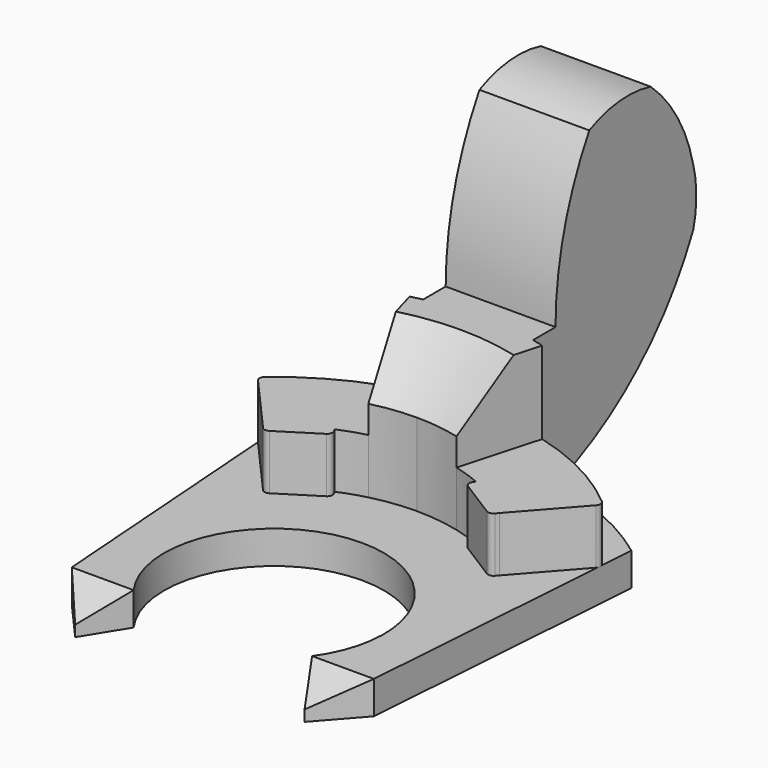
from build123d import *

# Parameters (mm, degrees)
F1_DEPTH    = 1.2
F3_DEPTH    = 12.5
F5_DEPTH    = 2
F6_DEPTH    = 5
F7_T2_ANGLE = 119.2786087223
F8_DEPTH    = 5
F10_DEPTH   = 4
F11_DEPTH   = 5


# Not quite as in the source:
# - a fillet or chamfer that OpenCascade refuses, or shapes differently, is made with other operations: its cross-section is extruded or revolved along the edge and cut away or added
# - a feature names something its author has since deleted; it is built from what else it names


with BuildPart() as f1:
    # F0 (on Top) → F1 (new body)
    with BuildSketch(Plane.XY):
        with BuildLine():
            ThreePointArc((-3.25, -2.3318447633), (0, 4), (3.25, -2.3318447633))
            Line((3.25, -2.3318447633), (4.1771243445, -3.8318447633))
            Line((4.1771243445, -3.8318447633), (5.5, -2.3318447633))
            Line((5.5, -2.3318447633), (6.2861850371, 8.4103434936))
            ThreePointArc((6.2861850371, 8.4103434936), (0, 10.5), (-6.2861850371, 8.4103434936))
            Line((-6.2861850371, 8.4103434936), (-5.5, -2.3318447633))
            Line((-5.5, -2.3318447633), (-4.1771243445, -3.8318447633))
            Line((-4.1771243445, -3.8318447633), (-3.25, -2.3318447633))
        make_face()
    extrude(amount=F1_DEPTH)

    # F2 (on Right) → F3 (cut, symmetric)
    with BuildSketch(Plane.YZ):
        Polygon((-3.8318447633, 0.4), (-2.3318447633, 1.2), (-3.8318447633, 1.2), align=None)
    extrude(amount=F3_DEPTH, both=True, mode=Mode.SUBTRACT)

    # F4 (on face) → F5 (join)
    with BuildSketch(Plane.XY.offset(1.2)):
        with BuildLine():
            Line((0, 9.4893432962), (0, 9.5))
            ThreePointArc((0, 9.5), (-1.0056504861, 9.4466219941), (-2, 9.2870878105))
            ThreePointArc((-2, 9.2870878105), (-2.207287093, 9.2400153511), (-2.4134691055, 9.1883168686))
            Line((-2.4134691055, 9.1883168686), (-1.6054997382, 6.2986006851))
            ThreePointArc((-1.6054997382, 6.2986006851), (-0.809041268, 6.4494536378), (0, 6.5))
            Line((0, 6.5), (0, 9.4893432962))
        make_face()
        with BuildLine():
            Line((0, 10.3126084432), (0, 9.5))
            ThreePointArc((0, 9.5), (1.0056504861, 9.4466219941), (2, 9.2870878105))
            Line((2, 9.2870878105), (2, 10.3126084432))
            Line((2, 10.3126084432), (0, 10.3126084432))
        make_face()
        with BuildLine():
            ThreePointArc((2, 9.2870878105), (1.0056504861, 9.4466219941), (0, 9.5))
            Line((0, 9.5), (0, 9.4893432962))
            Line((0, 9.4893432962), (0, 6.5))
            ThreePointArc((0, 6.5), (0.809041268, 6.4494536378), (1.6054997382, 6.2986006851))
            Line((1.6054997382, 6.2986006851), (2.4134691055, 9.1883168686))
            ThreePointArc((2.4134691055, 9.1883168686), (2.207287093, 9.2400153511), (2, 9.2870878105))
        make_face()
        with BuildLine():
            ThreePointArc((-2, 9.2870878105), (-1.0056504861, 9.4466219941), (0, 9.5))
            Line((0, 9.5), (0, 10.3126084432))
            Line((0, 10.3126084432), (-2, 10.3126084432))
            Line((-2, 10.3126084432), (-2, 9.2870878105))
        make_face()
        with BuildLine():
            Line((-1.6054997382, 6.2986006851), (-2.4134691055, 9.1883168686))
            ThreePointArc((-2.4134691055, 9.1883168686), (-4.3834961594, 8.4282240965), (-6.1369591907, 7.2517399217))
            ThreePointArc((-6.1369591907, 7.2517399217), (-6.2072372931, 7.1135226449), (-6.1576144754, 6.9666192642))
            Line((-6.1576144754, 6.9666192642), (-4.3047045796, 4.8702688306))
            Line((-4.3047045796, 4.8702688306), (-4.2185888433, 4.7728389657))
            ThreePointArc((-4.2185888433, 4.7728389657), (-4.0971505607, 4.7073203992), (-3.9621862374, 4.7360357341))
            Line((-3.9621862374, 4.7360357341), (-2.5827247856, 5.6044208159))
            ThreePointArc((-2.5827247856, 5.6044208159), (-2.4942501859, 5.7293355978), (-2.5200172859, 5.8802246764))
            Line((-2.5200172859, 5.8802246764), (-2.5753119947, 5.968062343))
            ThreePointArc((-2.5753119947, 5.968062343), (-2.096928846, 6.152470188), (-1.6054997382, 6.2986006851))
        make_face()
        with BuildLine():
            ThreePointArc((6.1369591907, 7.2517399217), (4.3834961594, 8.4282240965), (2.4134691055, 9.1883168686))
            Line((2.4134691055, 9.1883168686), (1.6054997382, 6.2986006851))
            ThreePointArc((1.6054997382, 6.2986006851), (2.096928846, 6.152470188), (2.5753119947, 5.968062343))
            Line((2.5753119947, 5.968062343), (2.5200172859, 5.8802246764))
            ThreePointArc((2.5200172859, 5.8802246764), (2.4942501859, 5.7293355978), (2.5827247856, 5.6044208159))
            Line((2.5827247856, 5.6044208159), (3.9621862374, 4.7360357341))
            ThreePointArc((3.9621862374, 4.7360357341), (4.0971505607, 4.7073203992), (4.2185888433, 4.7728389657))
            Line((4.2185888433, 4.7728389657), (4.3047045796, 4.8702688306))
            Line((4.3047045796, 4.8702688306), (6.1576144754, 6.9666192642))
            ThreePointArc((6.1576144754, 6.9666192642), (6.2072372931, 7.1135226449), (6.1369591907, 7.2517399217))
        make_face()
    extrude(amount=F5_DEPTH)

    # F4 (on face) → F6 (join)
    with BuildSketch(Plane.XY.offset(1.2)):
        with BuildLine():
            ThreePointArc((2, 9.2870878105), (1.0056504861, 9.4466219941), (0, 9.5))
            Line((0, 9.5), (0, 9.4893432962))
            Line((0, 9.4893432962), (0, 6.5))
            ThreePointArc((0, 6.5), (0.809041268, 6.4494536378), (1.6054997382, 6.2986006851))
            Line((1.6054997382, 6.2986006851), (2.4134691055, 9.1883168686))
            ThreePointArc((2.4134691055, 9.1883168686), (2.207287093, 9.2400153511), (2, 9.2870878105))
        make_face()
        with BuildLine():
            Line((0, 9.4893432962), (0, 9.5))
            ThreePointArc((0, 9.5), (-1.0056504861, 9.4466219941), (-2, 9.2870878105))
            ThreePointArc((-2, 9.2870878105), (-2.207287093, 9.2400153511), (-2.4134691055, 9.1883168686))
            Line((-2.4134691055, 9.1883168686), (-1.6054997382, 6.2986006851))
            ThreePointArc((-1.6054997382, 6.2986006851), (-0.809041268, 6.4494536378), (0, 6.5))
            Line((0, 6.5), (0, 9.4893432962))
        make_face()
    extrude(amount=F6_DEPTH)

    # F7: chamfer of 2 on 1 edges, made by hand

    # F7_s1 → F7_t2 (revolve, cut)
    with BuildSketch(Plane(origin=(0, 0, 0), x_dir=(0, 0, 1), z_dir=(-0.5054419689, -0.8628606006, 0))):
        Polygon((6.2, 8.5), (4.2, 6.5), (6.2, 6.5), align=None)
    revolve(axis=Axis((0, 0, 6.2), (0, 0, -1)), revolution_arc=F7_T2_ANGLE, mode=Mode.SUBTRACT)

    # F4 (on face) → F8 (join, through all)
    with BuildSketch(Plane.XY.offset(1.2)):
        with BuildLine():
            Line((0, 10.3126084432), (0, 9.5))
            ThreePointArc((0, 9.5), (1.0056504861, 9.4466219941), (2, 9.2870878105))
            Line((2, 9.2870878105), (2, 10.307764064))
            ThreePointArc((2, 10.307764064), (1.9874359165, 10.3101939108), (1.974868881, 10.3126084432))
            Line((1.974868881, 10.3126084432), (0, 10.3126084432))
        make_face()
        with BuildLine():
            ThreePointArc((1.974868881, 10.3126084432), (1.9874359165, 10.3101939108), (2, 10.307764064))
            Line((2, 10.307764064), (2, 10.3126084432))
            Line((2, 10.3126084432), (1.974868881, 10.3126084432))
        make_face()
        with BuildLine():
            Line((-2, 10.3126084432), (-2, 10.307764064))
            ThreePointArc((-2, 10.307764064), (-1.9874359165, 10.3101939108), (-1.974868881, 10.3126084432))
            Line((-1.974868881, 10.3126084432), (-2, 10.3126084432))
        make_face()
        with BuildLine():
            ThreePointArc((-2, 9.2870878105), (-1.0056504861, 9.4466219941), (0, 9.5))
            Line((0, 9.5), (0, 10.3126084432))
            Line((0, 10.3126084432), (-1.974868881, 10.3126084432))
            ThreePointArc((-1.974868881, 10.3126084432), (-1.9874359165, 10.3101939108), (-2, 10.307764064))
            Line((-2, 10.307764064), (-2, 9.2870878105))
        make_face()
    extrude(amount=F8_DEPTH)

    # F9 (on face) → F10 (join)
    with BuildSketch(Plane(origin=(-2, 0, 0), x_dir=(0, -1, 0), z_dir=(-1, 0, 0))):
        with BuildLine():
            Line((-10.4906475171, 1.2), (-10.3126084432, 1.2))
            Line((-10.3126084432, 1.2), (-10.3126084432, 6.2))
            ThreePointArc((-10.3126084432, 6.2), (-10.7033019047, 9.142871965), (-11.848315427, 11.8818646297))
            ThreePointArc((-11.848315427, 11.8818646297), (-13.2228522743, 12.2616673302), (-14.6442650052, 12.1468305588))
            ThreePointArc((-14.6442650052, 12.1468305588), (-15.8696799602, 10.6519801079), (-16.5821556002, 8.8551500812))
            ThreePointArc((-16.5821556002, 8.8551500812), (-16.7217466821, 7.8095628414), (-16.5821556002, 6.7639756016))
            ThreePointArc((-16.5821556002, 6.7639756016), (-14.0870903715, 3.3790869985), (-10.4906475171, 1.2))
        make_face()
    extrude(amount=-F10_DEPTH)

    # F4 (on face) → F11 (join, through all)
    with BuildSketch(Plane.XY.offset(1.2)):
        with BuildLine():
            Line((0, 10.3126084432), (0, 9.5))
            ThreePointArc((0, 9.5), (1.0056504861, 9.4466219941), (2, 9.2870878105))
            Line((2, 9.2870878105), (2, 10.307764064))
            ThreePointArc((2, 10.307764064), (1.9874359165, 10.3101939108), (1.974868881, 10.3126084432))
            Line((1.974868881, 10.3126084432), (0, 10.3126084432))
        make_face()
        with BuildLine():
            ThreePointArc((-2, 9.2870878105), (-1.0056504861, 9.4466219941), (0, 9.5))
            Line((0, 9.5), (0, 10.3126084432))
            Line((0, 10.3126084432), (-1.974868881, 10.3126084432))
            ThreePointArc((-1.974868881, 10.3126084432), (-1.9874359165, 10.3101939108), (-2, 10.307764064))
            Line((-2, 10.307764064), (-2, 9.2870878105))
        make_face()
    extrude(amount=F11_DEPTH)


solid = f1.part
